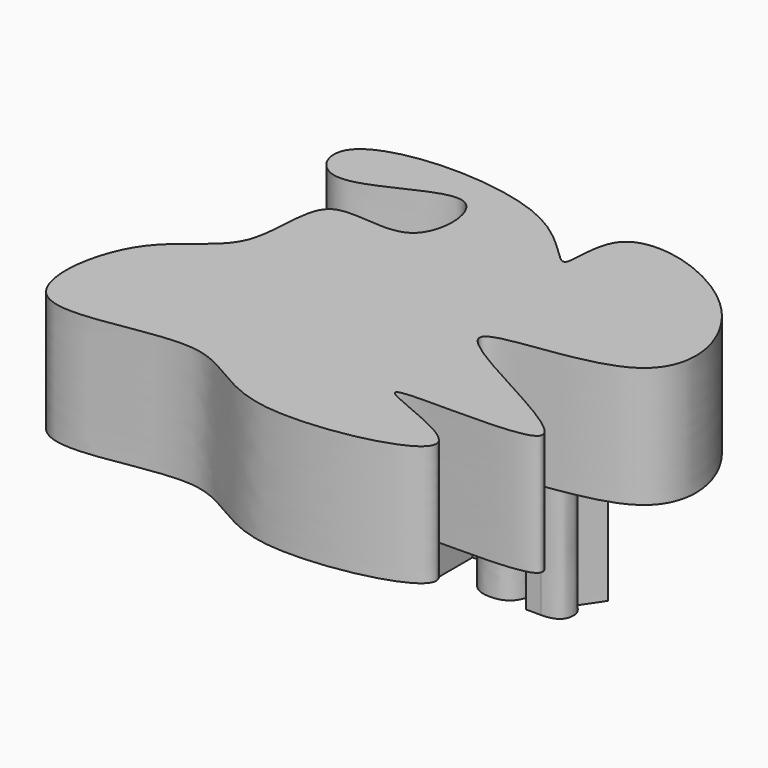
from build123d import *

# Parameters (mm, degrees)
F1_DEPTH     = 25.4
F2_TEXT_SIZE = 16.7325164916
F3_DEPTH     = 25.4
F4_TEXT_SIZE = 15.2021568889
F5_DEPTH     = 25.4


# Not quite as in the source:
# - Text() gives the source's letters only with a copy of the font that has no kerning and outlines rounded to 1/6400 em; it was checked with that copy


with BuildPart() as f1:
    # F0 (on Top) → F1 (new body)
    with BuildSketch(Plane.XY):
        with BuildLine():
            add(Edge.make_bspline(
                [(-38.9622151852, 34.7910784185), (-32.4980610606, 34.0209188821), (-13.5224458849, 50.4844086748), (-12.6279394629, 20.3597034293), (-37.9155505857, 31.3397770034), (-32.2711668457, 4.3727825842), (-51.9827489768, -0.9073241833), (-56.5653787073, -38.1069861085), (-15.5487512916, -21.1676506272), (-3.2548126842, -42.3622372201), (51.3493216579, -29.9258564749), (-3.4164776092, -15.3523596933), (72.4984376901, -22.5960493937), (-9.1383133718, 10.0799917286), (53.4421765311, 5.4406002904), (44.1743470769, 42.706212637), (7.4534713904, 53.3963297525), (11.6360576454, 27.4721208877), (-1.9473675341, 50.9811645867), (-50.512247402, 49.6594617312), (-43.1704963961, 35.2924662017), (-38.9622151852, 34.7910784185)],
                knots=[0, 0, 0, 0, 0.053087884, 0.0944446109, 0.1389559736, 0.1851778079, 0.2326467008, 0.2861154258, 0.3469528705, 0.4016942152, 0.4637561101, 0.5122346865, 0.5714577983, 0.6381198844, 0.6973159098, 0.7537677813, 0.8127404112, 0.8504261188, 0.8954645297, 0.9654388276, 1, 1, 1, 1], degree=3))
        make_face()
    extrude(amount=F1_DEPTH)

    # F2 (on face) → F3 (join)
    with BuildSketch(Plane(origin=(0, 0, 0), x_dir=(1, 0, 0), z_dir=(0, 0, -1))):
        with Locations((-8.1320609897, -27.0451679826)):
            Text('T', F2_TEXT_SIZE, font='Open Sans', font_style=FontStyle.BOLD, text_align=(TextAlign.LEFT, TextAlign.BOTTOM))
    extrude(amount=-F3_DEPTH)

    # F4 (on face) → F5 (join)
    with BuildSketch(Plane(origin=(0, 0, 0), x_dir=(1, 0, 0), z_dir=(0, 0, -1))):
        with Locations((-30.2116768435, -20.9153480828)):
            Text('TAYLOR', F4_TEXT_SIZE, font='Open Sans', font_style=FontStyle.BOLD, text_align=(TextAlign.LEFT, TextAlign.BOTTOM))
    extrude(amount=F5_DEPTH)


solid = f1.part
